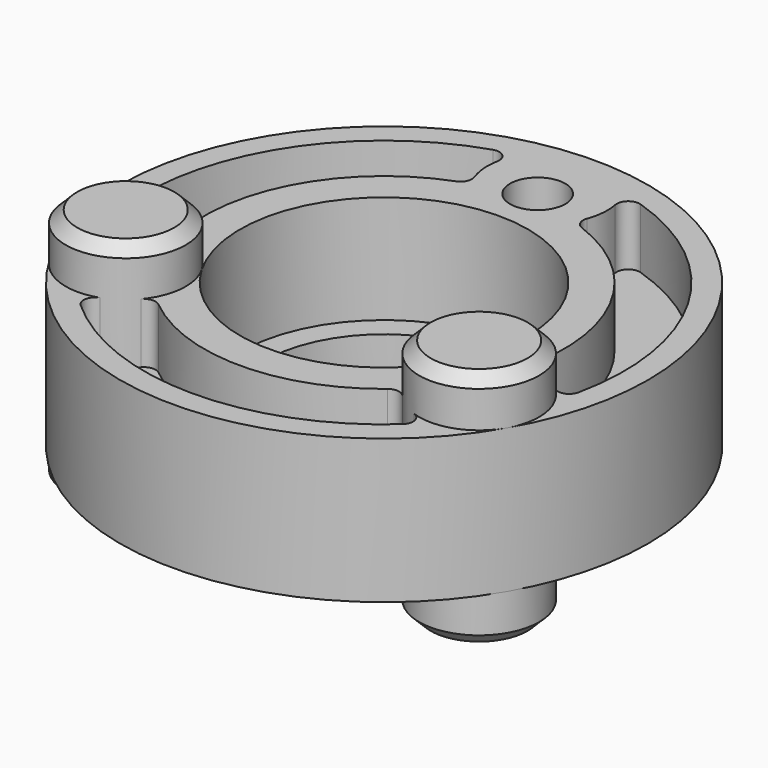
from build123d import *

# Parameters (mm, degrees)
F0_R            = 17.4625
F0_R_2          = 7.9375
F0_R_3          = 1.8288
F1_DEPTH        = 9.525
F2_R            = 9.525
F3_DEPTH        = 7.14375
F5_DEPTH        = 3.96875
F5_COPIES_COUNT = 3
F7_DEPTH        = 3.96875
F7_COPIES_COUNT = 3
F8_R            = 0.762
F10_R           = 3.96875
F11_DEPTH       = 3.175
F11_DEPTH_BACK  = 12.7
F12_SIZE        = 0.762


# Not quite as in the source:
# - a feature of the source that left no trace in its solid (it failed there, or was rolled back) is left out
# - a pattern or mirror of a feature is missing from the dataset's text; its kind, count and spacing are read off the source's solid


with BuildPart() as f1:
    # F0 (on Top) → F1 (new body)
    with BuildSketch(Plane.XY):
        Circle(F0_R)
        Circle(F0_R_2, mode=Mode.SUBTRACT)
        with Locations((0, 12.7)):
            Circle(F0_R_3, mode=Mode.SUBTRACT)
    extrude(amount=F1_DEPTH)

    # F2 (on face) → F3 (cut)
    with BuildSketch(Plane.XY.offset(9.525)):
        Circle(F2_R)
    extrude(amount=-F3_DEPTH, mode=Mode.SUBTRACT)

    # F4 (on face) → F5 (cut)
    with BuildSketch(Plane.XY.offset(9.525)):
        with BuildLine():
            ThreePointArc((-3.3814051731, 11.4159926471), (-3.9685398143, 13.4529051128), (-3.4234536074, 15.5014705882))
            ThreePointArc((-3.4234536074, 15.5014705882), (-13.7481532851, 7.9375), (-15.1363941291, -4.7859375014))
            ThreePointArc((-15.1363941291, -4.7859375014), (-13.6348274895, -3.2895962613), (-11.5772422283, -2.7796135431))
            ThreePointArc((-11.5772422283, -2.7796135431), (-10.3111149638, 5.953125), (-3.3814051731, 11.4159926471))
        make_face()
    f5 = extrude(amount=-F5_DEPTH, mode=Mode.SUBTRACT)

    # F5_copies: F5 ×3 about axis
    f5_copies_axis = Axis((0, 0, 0), (0, 0, 1))
    for i in range(1, F5_COPIES_COUNT):
        add(f5.rotate(f5_copies_axis, i * 360 / F5_COPIES_COUNT), mode=Mode.SUBTRACT)

    # F6 (on face) → F7 (cut)
    with BuildSketch(Plane(origin=(0, 0, 0), x_dir=(1, 0, 0), z_dir=(0, 0, -1))):
        with BuildLine():
            ThreePointArc((-11.5772422283, 2.7796135431), (-13.6348274895, 3.2895962613), (-15.1363941291, 4.7859375014))
            ThreePointArc((-15.1363941291, 4.7859375014), (-13.7481532851, -7.9375), (-3.4234536074, -15.5014705882))
            ThreePointArc((-3.4234536074, -15.5014705882), (-3.9685398143, -13.4529051128), (-3.3814051731, -11.4159926471))
            ThreePointArc((-3.3814051731, -11.4159926471), (-10.3111149638, -5.953125), (-11.5772422283, 2.7796135431))
        make_face()
    f7 = extrude(amount=-F7_DEPTH, mode=Mode.SUBTRACT)

    # F7_copies: F7 ×3 about axis
    f7_copies_axis = Axis((0, 0, 0), (0, 0, 1))
    for i in range(1, F7_COPIES_COUNT):
        add(f7.rotate(f7_copies_axis, i * 360 / F7_COPIES_COUNT), mode=Mode.SUBTRACT)

    # F8
    f8_edges = [f1.edges().sort_by_distance(p)[0] for p in [
        (-15.136394, -4.785938, 7.540625),
        (-11.577242, -2.779614, 7.540625),
        (-3.381405, 11.415993, 7.540625),
        (-3.423454, 15.501471, 7.540625),
        (-3.381405, 11.415993, 1.984375),
        (-3.423454, 15.501471, 1.984375),
        (-11.577242, -2.779614, 1.984375),
        (-15.136394, -4.785938, 1.984375),
        (8.195837, -8.636379, 1.984375),
        (11.712941, -10.715533, 1.984375),
        (-8.195837, -8.636379, 1.984375),
        (-11.712941, -10.715533, 1.984375),
        (3.381405, 11.415993, 1.984375),
        (3.423454, 15.501471, 1.984375),
        (11.577242, -2.779614, 1.984375),
        (15.136394, -4.785938, 1.984375),
        (11.712941, -10.715533, 7.540625),
        (8.195837, -8.636379, 7.540625),
        (-11.712941, -10.715533, 7.540625),
        (-8.195837, -8.636379, 7.540625),
        (3.423454, 15.501471, 7.540625),
        (3.381405, 11.415993, 7.540625),
        (11.577242, -2.779614, 7.540625),
        (15.136394, -4.785938, 7.540625),
    ]]
    fillet(f8_edges, radius=F8_R)

    # F10 (on face) → F11 (join, two sides)
    with BuildSketch(Plane(origin=(0, 0, 0), x_dir=(1, 0, 0), z_dir=(0, 0, -1))) as f11_sk:
        with Locations((11.6859302923, 6.746875)):
            Circle(F10_R)
        with Locations((-11.6859302923, 6.746875)):
            Circle(F10_R)
    extrude(amount=F11_DEPTH)
    extrude(f11_sk.sketch, amount=-F11_DEPTH_BACK)

    # F12
    f12_edges = [f1.edges().sort_by_distance(p)[0] for p in [
        (-15.65468, -6.746875, 12.7),
        (7.71718, -6.746875, 12.7),
        (7.71718, -6.746875, -3.175),
        (-15.65468, -6.746875, -3.175),
    ]]
    chamfer(f12_edges, length=F12_SIZE)


solid = f1.part
